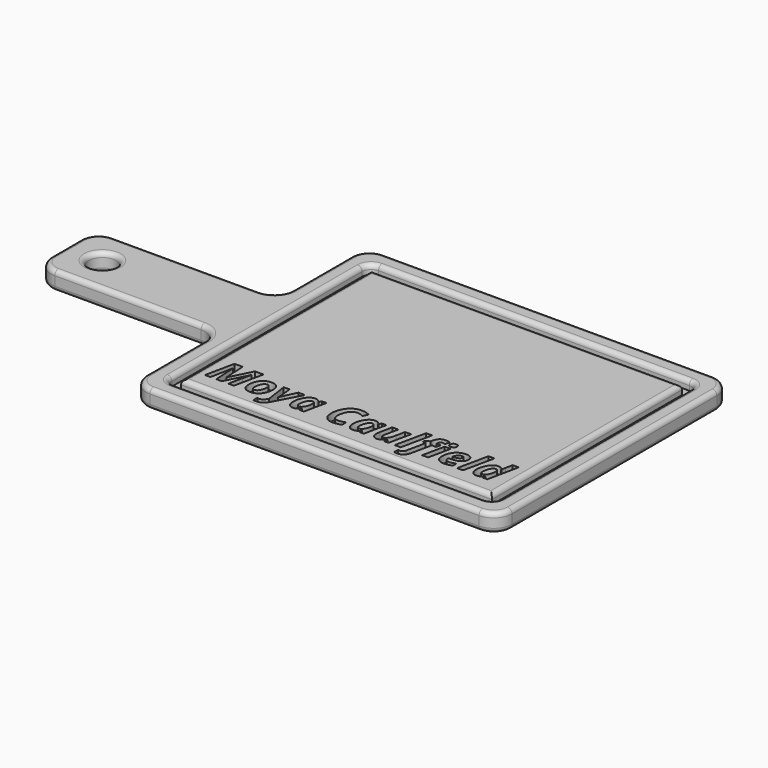
from build123d import *

# Parameters (mm, degrees)
F0_W         = 127
F0_H         = 50.8
F1_DEPTH     = 12.7
F2_R         = 9.525
F3_DEPTH     = 25.4
F5_DEPTH     = 6.35
F6_R         = 6.35
F7_R         = 12.7
F8_R         = 3.175
F9_TEXT_SIZE = 28.3959998253
F10_DEPTH    = 5.08


# Not quite as in the source:
# - Text() gives the source's letters only with a copy of the font that has no kerning and outlines rounded to 1/6400 em; it was checked with that copy


with BuildPart() as f1:
    # F0 (on Top) → F1 (new body)
    with BuildSketch(Plane.XY):
        Polygon((0, 76.2), (0, 0), (254, 0), (254, 203.2), (0, 203.2), (0, 127), align=None)
        with Locations((-63.5, 101.6)):
            Rectangle(F0_W, F0_H)
    extrude(amount=F1_DEPTH)

    # F2 (on face) → F3 (cut)
    with BuildSketch(Plane.XY.offset(12.7)):
        with Locations((-101.6, 101.6)):
            Circle(F2_R)
    extrude(amount=-F3_DEPTH, mode=Mode.SUBTRACT)

    # F4 (on face) → F5 (cut)
    with BuildSketch(Plane.XY.offset(12.7)):
        Polygon((12.6999939203, 76.2), (12.6999939203, 12.6999939203), (241.3000060797, 12.6999939203), (241.3000060797, 190.5000060797), (12.6999939203, 190.5000060797), (12.6999939203, 127), align=None)
        Polygon((19.0499939203, 76.2), (19.0499939203, 127), (19.0499939203, 184.1500060797), (234.9500060797, 184.1500060797), (234.9500060797, 19.0499939203), (19.0499939203, 19.0499939203), align=None, mode=Mode.SUBTRACT)
    extrude(amount=-F5_DEPTH, mode=Mode.SUBTRACT)

    # F6
    f6_edges = [f1.edges().sort_by_distance(p)[0] for p in [
        (12.699994, 12.699994, 9.525),
        (12.699994, 190.500006, 9.525),
        (241.300006, 12.699994, 9.525),
        (241.300006, 190.500006, 9.525),
    ]]
    fillet(f6_edges, radius=F6_R)

    # F7
    f7_edges = [f1.edges().sort_by_distance(p)[0] for p in [
        (254, 203.2, 6.35),
        (0, 203.2, 6.35),
        (-127, 127, 6.35),
        (-127, 76.2, 6.35),
        (0, 0, 6.35),
        (254, 0, 6.35),
        (0, 127, 6.35),
        (0, 76.2, 6.35),
    ]]
    fillet(f7_edges, radius=F7_R)

    # F8
    f8_edges = [f1.edges().sort_by_distance(p)[0] for p in [
        (127, 19.049994, 12.7),
        (19.049994, 101.6, 12.7),
        (127, 184.150006, 12.7),
        (234.950006, 101.6, 12.7),
        (0, 38.1, 12.7),
        (-3.719744, 72.480256, 12.7),
        (3.719744, 3.719744, 12.7),
        (-63.5, 76.2, 12.7),
        (127, 0, 12.7),
        (-123.280256, 79.919744, 12.7),
        (250.280256, 3.719744, 12.7),
        (-127, 101.6, 12.7),
        (254, 101.6, 12.7),
        (-123.280256, 123.280256, 12.7),
        (250.280256, 199.480256, 12.7),
        (-63.5, 127, 12.7),
        (127, 203.2, 12.7),
        (-3.719744, 130.719744, 12.7),
        (3.719744, 199.480256, 12.7),
        (0, 165.1, 12.7),
        (127, 12.699994, 12.7),
        (14.559866, 14.559866, 12.7),
        (239.440134, 14.559866, 12.7),
        (12.699994, 101.6, 12.7),
        (241.300006, 101.6, 12.7),
        (14.559866, 188.640134, 12.7),
        (239.440134, 188.640134, 12.7),
        (127, 190.500006, 12.7),
        (-111.125, 101.6, 12.7),
        (0, 38.1, 0),
        (-3.719744, 72.480256, 0),
        (3.719744, 3.719744, 0),
        (-63.5, 76.2, 0),
        (127, 0, 0),
        (-123.280256, 79.919744, 0),
        (250.280256, 3.719744, 0),
        (-127, 101.6, 0),
        (254, 101.6, 0),
        (-123.280256, 123.280256, 0),
        (250.280256, 199.480256, 0),
        (-63.5, 127, 0),
        (127, 203.2, 0),
        (-3.719744, 130.719744, 0),
        (3.719744, 199.480256, 0),
        (0, 165.1, 0),
        (-111.125, 101.6, 0),
    ]]
    fillet(f8_edges, radius=F8_R)

    # F9 (on face) → F10 (cut)
    with BuildSketch(Plane.XY.offset(12.7)):
        with Locations((25.1410562484, 31.3113110314)):
            Text('Moya Caulfield', F9_TEXT_SIZE, font='Open Sans', font_style=FontStyle.BOLDITALIC, text_align=(TextAlign.LEFT, TextAlign.BOTTOM))
    extrude(amount=-F10_DEPTH, mode=Mode.SUBTRACT)


solid = f1.part
